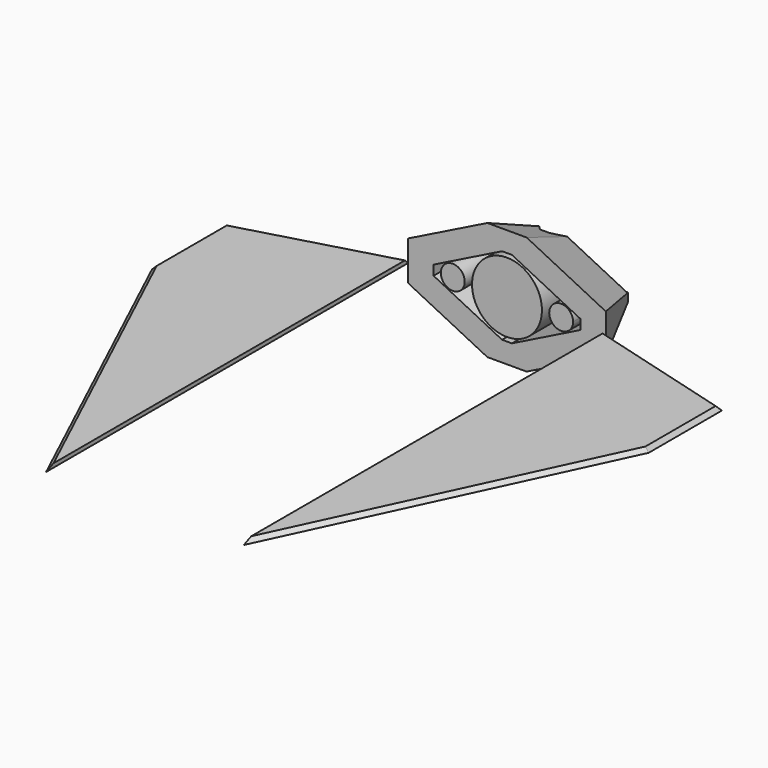
from build123d import *

# Parameters (mm, degrees)
F1_DEPTH         = 2.54
F1_DEPTH_BACK    = 2.54
F2_SIZE          = 5.07999
F5_DEPTH         = 76.2
F6_T1_DEPTH      = 509.1856975688
F6_T3_DEPTH      = 445.8733729354
F6_T5_DEPTH      = 509.1856975688
F6_T7_DEPTH      = 445.8733729354
F6_T9_DEPTH      = 509.1856975688
F6_T11_DEPTH     = 509.1856975688
F4_R             = 45.1305930008
F7_DEPTH         = 82.55
F8_DEPTH         = 76.2
F4_R_2           = 15.4174158708
F9_SIZE          = 12.7
F10_R            = 10.16
F12_D            = 63.5
F12_DEPTH        = 25.4
F12_START        = 0.6321404
F12_TIP          = 19.0773246541
F13_SIZE         = 5.08
F15_R            = 7.62
F15_2_R          = 7.62
F18_D            = 19.05
F18_DEPTH        = 19.05
F18_TIP          = 5.7231973962
F18_ON_F17_D     = 19.05
F18_ON_F17_DEPTH = 19.05
F18_ON_F17_TIP   = 5.7231973962


# Not quite as in the source:
# - a fillet or chamfer that OpenCascade refuses, or shapes differently, is made with other operations: its cross-section is extruded or revolved along the edge and cut away or added
# - a fillet or chamfer is up to 0.001 mm smaller than in the source, because OpenCascade refuses the exact size


with BuildPart() as f1:
    # F0 (on Top) → F1 (new body, two sides)
    with BuildSketch(Plane.XY) as f1_sk:
        Polygon((320.5616772175, -53.8842752576), (127.5811266, 0), (127.5811266, -584.2), (320.5616772175, -172.0790863037), align=None)
    extrude(amount=F1_DEPTH)
    extrude(f1_sk.sketch, amount=-F1_DEPTH_BACK)

    # F2 (size 5.08 in the source; OpenCascade refuses exactly that, so slightly less here)
    f2_edges = [f1.edges().sort_by_distance(p)[0] for p in [
        (224.071402, -378.139543, 2.54),
        (320.561677, -112.981681, 2.54),
        (224.071402, -26.942138, 2.54),
    ]]
    chamfer(f2_edges, length=F2_SIZE)


with BuildPart() as f3_1:
    # F3: instance of F1
    add(f1.part.mirror(Plane.YZ))


with BuildPart() as f5:
    # F4 (on Front) → F5 (new body)
    with BuildSketch(Plane.XZ):
        Polygon((-127.5811266, 25.4), (-127.5811266, 0), (-127.5811266, -25.4), (-25.4, -76.2), (0, -76.2), (25.4, -76.2), (127.5811266, -25.4), (127.5811266, 0), (127.5811266, 25.4), (25.4, 76.2), (0, 76.2), (-25.4, 76.2), align=None)
        Polygon((94.7542563081, 6.35), (94.7542563081, 0), (94.7542563081, -6.35), (6.35, -50.3007409038), (-6.35, -50.3007409038), (-94.7542563081, -6.35), (-94.7542563081, 6.35), (-6.35, 50.3007409038), (6.35, 50.3007409038), align=None, mode=Mode.SUBTRACT)
    extrude(amount=-F5_DEPTH)

    # F6: chamfer of 76.2 x 32.3449809952 on 8 edges, made by hand

    # F6_s2 → F6_t1 (cut)
    with BuildSketch(Plane(origin=(269.0546874739, 0, -133.7622570671), x_dir=(0, 1, 0), z_dir=(-0.8954433882, 0, 0.4451754021))):
        Polygon((0, -79.54024139), (76.2, -47.1952603949), (76.2, -79.54024139), align=None)
    extrude(amount=F6_T1_DEPTH, mode=Mode.SUBTRACT)

    # F6_s4 → F6_t3 (cut)
    with BuildSketch(Plane.YZ.offset(-222.9366864677)):
        Polygon((76.2, 43.8550190048), (0, 76.2), (76.2, 76.2), align=None)
        Polygon((76.2, -43.8550190048), (0, -76.2), (76.2, -76.2), align=None)
    extrude(amount=F6_T3_DEPTH, mode=Mode.SUBTRACT)

    # F6_s6 → F6_t5 (cut)
    with BuildSketch(Plane(origin=(186.8922787572, 0, 92.9146905772), x_dir=(0, 1, 0), z_dir=(-0.8954433882, 0, -0.4451754021))):
        Polygon((76.2, -47.1952603949), (0, -79.54024139), (76.2, -79.54024139), align=None)
    extrude(amount=F6_T5_DEPTH, mode=Mode.SUBTRACT)

    # F6_s8 → F6_t7 (cut)
    with BuildSketch(Plane.XY.offset(-222.9366864677)):
        Polygon((-95.2361456048, 76.2), (-127.5811266, 0), (-127.5811266, 76.2), align=None)
        Polygon((95.2361456048, 76.2), (127.5811266, 0), (127.5811266, 76.2), align=None)
    extrude(amount=F6_T7_DEPTH, mode=Mode.SUBTRACT)

    # F6_s10 → F6_t9 (cut)
    with BuildSketch(Plane(origin=(-269.0546874739, 0, 133.7622570671), x_dir=(0, 1, 0), z_dir=(0.8954433882, 0, -0.4451754021))):
        Polygon((76.2, -47.1952603949), (0, -79.54024139), (76.2, -79.54024139), align=None)
    extrude(amount=F6_T9_DEPTH, mode=Mode.SUBTRACT)

    # F6_s12 → F6_t11 (cut)
    with BuildSketch(Plane(origin=(-186.8922787572, 0, -92.9146905772), x_dir=(0, 1, 0), z_dir=(0.8954433882, 0, 0.4451754021))):
        Polygon((76.2, -47.1952603949), (0, -79.54024139), (76.2, -79.54024139), align=None)
    extrude(amount=F6_T11_DEPTH, mode=Mode.SUBTRACT)


with BuildPart() as f7:
    # F4 (on Front) → F7 (new body)
    with BuildSketch(Plane.XZ):
        Circle(F4_R)
    extrude(amount=-F7_DEPTH)

    # F9
    f9_edges = [f7.edges().sort_by_distance(p)[0] for p in [
        (-45.130593, 82.55, 0),
    ]]
    chamfer(f9_edges, length=F9_SIZE)

    # F10
    f10_edges = [f7.edges().sort_by_distance(p)[0] for p in [
        (-32.430593, 82.55, 0),
    ]]
    fillet(f10_edges, radius=F10_R)

    # F12
    # its depths count from where the whole tool has entered the part; down to there all is cleared
    with Locations(Plane(origin=(0, 82.55, 0), x_dir=(-1, 0, 0), z_dir=(0, 1, 0)).offset(-F12_START)):
        with Locations((0, 0)):
            Hole(F12_D / 2, depth=F12_DEPTH)
            with Locations((0, 0, -(F12_DEPTH + F12_TIP / 2))):  # 118° drill point
                Cone(0, F12_D / 2, F12_TIP, mode=Mode.SUBTRACT)

    # F13
    f13_edges = [f7.edges().sort_by_distance(p)[0] for p in [
        (-45.130593, 69.85, 0),
    ]]
    chamfer(f13_edges, length=F13_SIZE)


with BuildPart() as f8:
    # F4 (on Front) → F8 (new body)
    with BuildSketch(Plane.XZ):
        with BuildLine():
            Line((54.5250087836, 0), (85.3598405253, 0))
            ThreePointArc((85.3598405253, 0), (69.9424246545, 15.4174158708), (54.5250087836, 0))
        make_face()
        with BuildLine():
            ThreePointArc((54.5250087836, 0), (69.9424246545, -15.4174158708), (85.3598405253, 0))
            Line((85.3598405253, 0), (54.5250087836, 0))
        make_face()
    extrude(amount=-F8_DEPTH)

    # F14: chamfer of 5.08 on 1 edges, made by hand

    # F14_s1 → F14_t2 (revolve, cut)
    with BuildSketch(Plane.XY):
        Polygon((54.5250087836, 71.12), (59.6050087836, 76.2), (54.5250087836, 76.2), align=None)
    revolve(axis=Axis((69.9424246545, 76.2, 0), (0, -1, 0)), mode=Mode.SUBTRACT)

    # F15
    f15_edges = [f8.edges().sort_by_distance(p)[0] for p in [
        (85.359841, 71.12, 0),
    ]]
    fillet(f15_edges, radius=F15_R)

    # F18
    with Locations(Plane(origin=(0, 76.2, 0), x_dir=(-1, 0, 0), z_dir=(0, 1, 0))):
        with Locations((-69.9424246545, 0)):
            Hole(F18_D / 2, depth=F18_DEPTH)
            with Locations((0, 0, -(F18_DEPTH + F18_TIP / 2))):  # 118° drill point
                Cone(0, F18_D / 2, F18_TIP, mode=Mode.SUBTRACT)


with BuildPart() as f8b:
    # F4 (on Front) → F8, piece 2 (new body)
    with BuildSketch(Plane.XZ):
        with Locations((-69.9424246545, 0)):
            Circle(F4_R_2)
    extrude(amount=-F8_DEPTH)

    # F14#2: chamfer of 5.08 on 1 edges, made by hand

    # F14_2_s1 → F14_2_t2 (revolve, cut)
    with BuildSketch(Plane.XY):
        Polygon((-54.5250087836, 71.12), (-59.6050087836, 76.2), (-54.5250087836, 76.2), align=None)
    revolve(axis=Axis((-69.9424246545, 76.2, 0), (0, -1, 0)), mode=Mode.SUBTRACT)

    # F15#2
    f15_2_edges = [f8b.edges().sort_by_distance(p)[0] for p in [
        (-85.359841, 71.12, 0),
    ]]
    fillet(f15_2_edges, radius=F15_2_R)

    # F18 on F17
    with Locations(Plane(origin=(0, 76.2, 0), x_dir=(-1, 0, 0), z_dir=(0, 1, 0))):
        with Locations((69.9424246545, 0)):
            Hole(F18_ON_F17_D / 2, depth=F18_ON_F17_DEPTH)
            with Locations((0, 0, -(F18_ON_F17_DEPTH + F18_ON_F17_TIP / 2))):  # 118° drill point
                Cone(0, F18_ON_F17_D / 2, F18_ON_F17_TIP, mode=Mode.SUBTRACT)


solid = Compound([f1.part, f3_1.part, f5.part, f7.part, f8.part, f8b.part])
